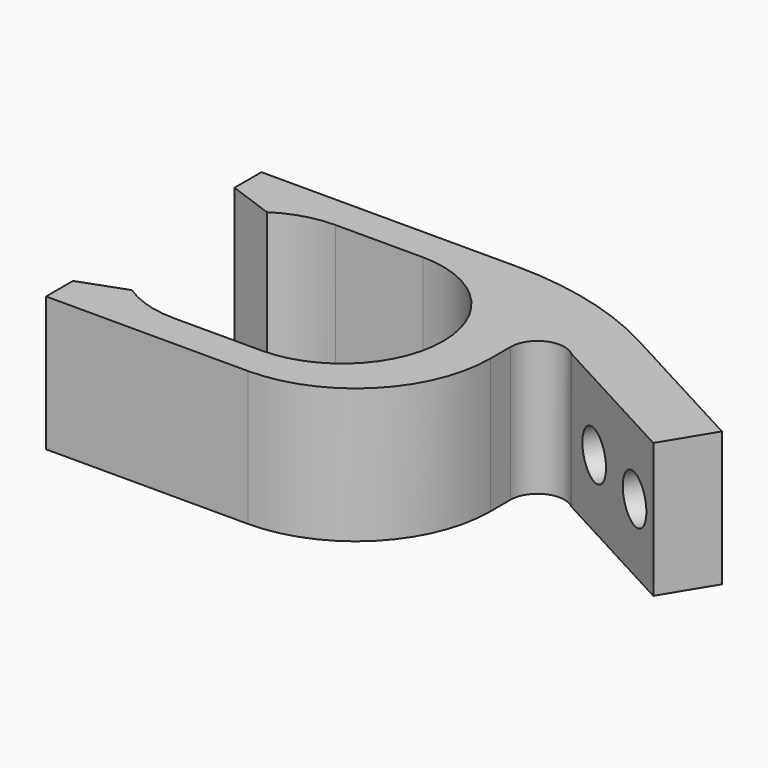
from build123d import *

# Parameters (mm, degrees)
F1_DEPTH = 5
F2_R     = 1.75
F3_DEPTH = 9.9
F4_R     = 24


# Not quite as in the source:
# - a feature names something its author has since deleted; it is built from what else it names


with BuildPart() as f1:
    # F0 (on Top) → F1 (new body, symmetric)
    with BuildSketch(Plane.XY):
        with BuildLine():
            Line((16.2096246684, 11.2512872423), (0, 20))
            Line((0, 20), (-25, 20))
            Line((-25, 20), (-25, 17.5))
            Line((-25, 17.5), (-17.5, 17.5))
            Line((-17.5, 17.5), (-11, 17.5))
            Line((-11, 17.5), (-3.5, 17.5))
            Line((-3.5, 17.5), (-3.5, 10))
            Line((-3.5, 10), (-3.5, 2.5))
            Line((-3.5, 2.5), (-11, 2.5))
            Line((-11, 2.5), (-17.5, 2.5))
            Line((-17.5, 2.5), (-25, 2.5))
            Line((-25, 2.5), (-25, 0))
            Line((-25, 0), (-10, 0))
            ThreePointArc((-10, 0), (-2.9289321881, 2.9289321881), (0, 10))
            Line((0, 10), (0, 11.8892861952))
            ThreePointArc((0, 11.8892861952), (1.1623016269, 13.7053978206), (3.2982614357, 13.4106399491))
            Line((3.2982614357, 13.4106399491), (14.0066361954, 7.6310801635))
            Line((14.0066361954, 7.6310801635), (16.2096246684, 11.2512872423))
        make_face()
        with BuildLine():
            Line((-17.5, 17.5), (-25, 17.5))
            Line((-25, 17.5), (-21.614659653, 16.270532349))
            ThreePointArc((-21.614659653, 16.270532349), (-19.6472083483, 17.186062643), (-17.5, 17.5))
        make_face()
        with BuildLine():
            Line((-21.614659653, 3.729467651), (-25, 2.5))
            Line((-25, 2.5), (-17.5, 2.5))
            ThreePointArc((-17.5, 2.5), (-19.6472083483, 2.813937357), (-21.614659653, 3.729467651))
        make_face()
        with BuildLine():
            Line((-3.5, 17.5), (-11, 17.5))
            ThreePointArc((-11, 17.5), (-5.6966991411, 15.3033008589), (-3.5, 10))
            Line((-3.5, 10), (-3.5, 17.5))
        make_face()
        with BuildLine():
            Line((-3.5, 2.5), (-3.5, 10))
            ThreePointArc((-3.5, 10), (-5.6966991411, 4.6966991411), (-11, 2.5))
            Line((-11, 2.5), (-3.5, 2.5))
        make_face()
    extrude(amount=F1_DEPTH, both=True)

    # F2 (on face) → F3 (cut)
    with BuildSketch(Plane(origin=(8.3593712251, 15.4882522465, 0), x_dir=(-0.8800071661, 0.4749604064, 0), z_dir=(0.4749604064, 0.8800071661, 0))):
        with Locations((-5.9206699059, 0)):
            Circle(F2_R)
        with Locations((0.0793300941, 0)):
            Circle(F2_R)
    extrude(amount=-F3_DEPTH, mode=Mode.SUBTRACT)

    # F4
    f4_edges = [f1.edges().sort_by_distance(p)[0] for p in [
        (0, 20, 0),
    ]]
    fillet(f4_edges, radius=F4_R)


solid = f1.part
